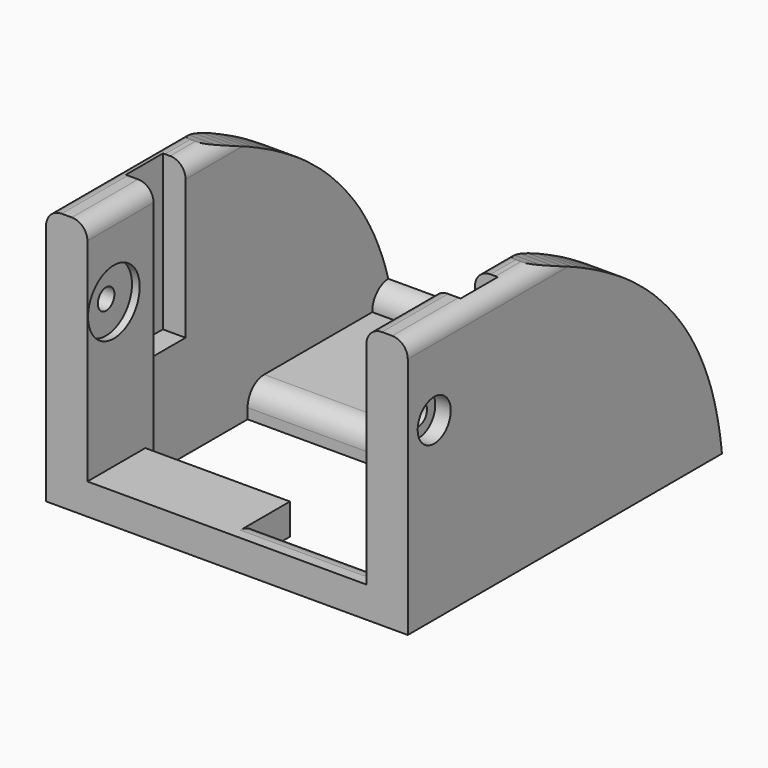
from build123d import *

# Parameters (mm, degrees)
F0_W         = 28
F0_H         = 18
F1_DEPTH     = 3
F2_DEPTH     = 25
F3_R         = 2
F4_R         = 1
F5_DEPTH     = 50
F0_W_2       = 2.2
F0_H_2       = 4.5
F6_DEPTH     = 10
F9_DEPTH     = 100
F4_R_2       = 3.125
F10_R        = 3.125
F10_R_2      = 1
F11_DEPTH    = 0.75
F12_T1_DEPTH = 25.6433879336
F12_T3_DEPTH = 13.1433879336
F12_T5_DEPTH = 15.5
F13_DEPTH    = 35
F14_DEPTH    = 39
F15_T1_DEPTH = 28
F7_R         = 2
F7_R_2       = 1
F8_R         = 2
F8_R_2       = 1
F16_DEPTH    = 1.5


# Not quite as in the source:
# - a fillet or chamfer that OpenCascade refuses, or shapes differently, is made with other operations: its cross-section is extruded or revolved along the edge and cut away or added


with BuildPart() as f1:
    # F0 (on Top) → F1 (new body)
    with BuildSketch(Plane.XY):
        Polygon((-17.5, 0), (-17.5, -7), (-13.5, -7), (-13.5, 0), (-13.5, 1), (-14, 1), (-16.2, 1), (-16.2, 5.5), (-14, 5.5), (-14, 13), (-14, 31), (-17.5, 31), align=None)
        Polygon((-13.5, 0), (-13.5, -7), (13.5, -7), (13.5, 0), (12.5, 0), (12.5, -4), (0.5, -4), (0.5, 0), align=None)
        Polygon((13.5, 0), (13.5, -7), (17.5, -7), (17.5, 0), (17.5, 31), (14, 31), (14, 13), (14, 5.5), (16.2, 5.5), (16.2, 1), (14, 1), (13.5, 1), align=None)
        with Locations((0, 22)):
            Rectangle(F0_W, F0_H)
    extrude(amount=F1_DEPTH)

    # F0 (on Top) → F2 (join)
    with BuildSketch(Plane.XY):
        Polygon((-17.5, 0), (-17.5, -7), (-13.5, -7), (-13.5, 0), (-13.5, 1), (-14, 1), (-16.2, 1), (-16.2, 5.5), (-14, 5.5), (-14, 13), (-14, 31), (-17.5, 31), align=None)
        Polygon((13.5, 0), (13.5, -7), (17.5, -7), (17.5, 0), (17.5, 31), (14, 31), (14, 13), (14, 5.5), (16.2, 5.5), (16.2, 1), (14, 1), (13.5, 1), align=None)
    extrude(amount=F2_DEPTH)

    # F3
    f3_edges = [f1.edges().sort_by_distance(p)[0] for p in [
        (0, 13, 3),
        (6.5, -4, 3),
    ]]
    fillet(f3_edges, radius=F3_R)

    # F4 (on face) → F5 (cut, symmetric)
    with BuildSketch(Plane(origin=(13.5, 0, 0), x_dir=(0, -1, 0), z_dir=(-1, 0, 0))):
        with Locations((3.8, 17)):
            Circle(F4_R)
    extrude(amount=F5_DEPTH, both=True, mode=Mode.SUBTRACT)

    # F0 (on Top) → F6 (join)
    with BuildSketch(Plane.XY):
        with Locations((15.1, 3.25)):
            Rectangle(F0_W_2, F0_H_2)
        with Locations((-15.1, 3.25)):
            Rectangle(F0_W_2, F0_H_2)
    extrude(amount=F6_DEPTH)

    # F7 (on face) → F9 (cut)
    with BuildSketch(Plane(origin=(-17.5, 0, 0), x_dir=(0, -1, 0), z_dir=(-1, 0, 0))):
        Polygon((-31, 25), (-31, 3), (-30.5205184888, 3), (-30.311506, 3.940513), (-30.015185, 5.062344), (-29.67651, 6.184174), (-29.274339, 7.284839), (-28.829835, 8.364339), (-28.343022, 9.422672), (-27.792668, 10.459839), (-27.200003, 11.475841), (-26.565008, 12.470677), (-25.88768, 13.402016), (-25.146834, 14.333332), (-24.384844, 15.222339), (-23.580522, 16.069015), (-22.755012, 16.894503), (-21.887171, 17.67768), (-20.97702, 18.418505), (-20.066847, 19.138164), (-19.114343, 19.815513), (-18.119507, 20.450509), (-17.124671, 21.064339), (-16.108669, 21.657003), (-15.071502, 22.207335), (-14.034334, 22.736502), (-12.976001, 23.244503), (-11.896502, 23.710172), (-10.817003, 24.154675), (-9.737503, 24.556847), (-8.636839, 24.958997), (-8.5183879336, 25), align=None)
    extrude(amount=-F9_DEPTH, mode=Mode.SUBTRACT)

    # F4 (on face) + F10 (on face) → F11 (cut, symmetric)
    with BuildSketch(Plane(origin=(13.5, 0, 0), x_dir=(0, -1, 0), z_dir=(-1, 0, 0))):
        with Locations((3.8, 17)):
            Circle(F4_R_2)
        with Locations((3.8, 17)):
            Circle(F4_R, mode=Mode.SUBTRACT)
    with BuildSketch(Plane.YZ.offset(-13.5)):
        with Locations((-3.8, 17)):
            Circle(F10_R)
        with Locations((-3.8, 17)):
            Circle(F10_R_2, mode=Mode.SUBTRACT)
    extrude(amount=F11_DEPTH, both=True, dir=(-1, 0, 0), mode=Mode.SUBTRACT)

    # F12: fillet of radius 1.5 on 6 edges, made by hand

    # F12_s2 → F12_t1 (cut)
    with BuildSketch(Plane.XZ.offset(-14.8933879336)):
        with BuildLine():
            ThreePointArc((16, 25), (17.0606601718, 24.5606601718), (17.5, 23.5))
            Line((17.5, 23.5), (17.5, 25))
            Line((17.5, 25), (16, 25))
        make_face()
        with BuildLine():
            ThreePointArc((-17.5, 23.5), (-17.0606601718, 24.5606601718), (-16, 25))
            Line((-16, 25), (-17.5, 25))
            Line((-17.5, 25), (-17.5, 23.5))
        make_face()
    extrude(amount=F12_T1_DEPTH, mode=Mode.SUBTRACT)

    # F12_s4 → F12_t3 (cut)
    with BuildSketch(Plane.XZ.offset(-14.8933879336)):
        with BuildLine():
            ThreePointArc((15.5, 25), (14.4393398282, 24.5606601718), (14, 23.5))
            Line((14, 23.5), (14, 25))
            Line((14, 25), (15.5, 25))
        make_face()
        with BuildLine():
            ThreePointArc((-14, 23.5), (-14.4393398282, 24.5606601718), (-15.5, 25))
            Line((-15.5, 25), (-14, 25))
            Line((-14, 25), (-14, 23.5))
        make_face()
    extrude(amount=F12_T3_DEPTH, mode=Mode.SUBTRACT)

    # F12_s6 → F12_t5 (cut)
    with BuildSketch(Plane.XZ.offset(-4.75)):
        with BuildLine():
            ThreePointArc((13.5, 23.5), (13.9393398282, 24.5606601718), (15, 25))
            Line((15, 25), (13.5, 25))
            Line((13.5, 25), (13.5, 23.5))
        make_face()
        with BuildLine():
            ThreePointArc((-13.5, 23.5), (-13.9393398282, 24.5606601718), (-15, 25))
            Line((-15, 25), (-13.5, 25))
            Line((-13.5, 25), (-13.5, 23.5))
        make_face()
    extrude(amount=F12_T5_DEPTH, mode=Mode.SUBTRACT)

    # F7 (on face) → F13 (join)
    with BuildSketch(Plane(origin=(-17.5, 0, 0), x_dir=(0, -1, 0), z_dir=(-1, 0, 0))):
        Polygon((-30.311506, 3.940513), (-30.5205184888, 3), (-28.0815777779, 3), (-28.0815777779, 5.062344), (-30.015185, 5.062344), align=None)
    extrude(amount=-F13_DEPTH)

    # F7 (on face) → F14 (cut)
    with BuildSketch(Plane(origin=(-17.5, 0, 0), x_dir=(0, -1, 0), z_dir=(-1, 0, 0))):
        Polygon((-31, 3), (-31, 0), (-30.946502, 0.490336), (-30.777175, 1.654498), (-30.565517, 2.797516), (-30.5205184888, 3), align=None)
    extrude(amount=-F14_DEPTH, mode=Mode.SUBTRACT)

    # F15: fillet of radius 2 on 1 edges, made by hand

    # F15_s2 → F15_t1 (cut)
    with BuildSketch(Plane.YZ.offset(-14)):
        with BuildLine():
            ThreePointArc((28.0815777779, 3.063446304), (28.6440824638, 4.4539883645), (30.015185, 5.062344))
            Line((30.015185, 5.062344), (28.0815777779, 5.062344))
            Line((28.0815777779, 5.062344), (28.0815777779, 3.063446304))
        make_face()
    extrude(amount=F15_T1_DEPTH, mode=Mode.SUBTRACT)

    # F7 (on face) + F8 (on face) → F16 (cut, symmetric)
    with BuildSketch(Plane(origin=(-17.5, 0, 0), x_dir=(0, -1, 0), z_dir=(-1, 0, 0))):
        with Locations((3.8, 17)):
            Circle(F7_R)
        with Locations((3.8, 17)):
            Circle(F7_R_2, mode=Mode.SUBTRACT)
    with BuildSketch(Plane.YZ.offset(17.5)):
        with Locations((-3.8, 17)):
            Circle(F8_R)
        with Locations((-3.8, 17)):
            Circle(F8_R_2, mode=Mode.SUBTRACT)
    extrude(amount=F16_DEPTH, both=True, dir=(-1, 0, 0), mode=Mode.SUBTRACT)


solid = f1.part
